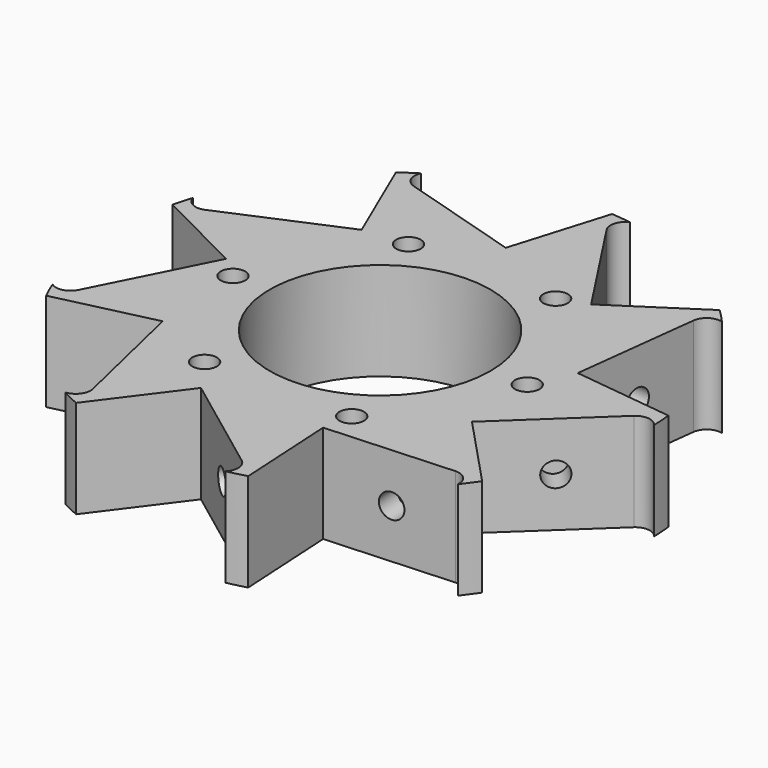
from build123d import *

# Parameters (mm, degrees)
F0_R      = 22.5
F1_DEPTH  = 20
F2_R      = 2.5
F3_DEPTH  = 20.001
F4_R      = 2.5
F5_DEPTH  = 5
F6_R      = 2.5
F7_DEPTH  = 5
F8_R      = 2.5
F9_DEPTH  = 5
F10_R     = 2.5
F11_DEPTH = 5
F12_R     = 2.5
F13_DEPTH = 5
F14_R     = 2.5
F15_DEPTH = 5
F16_R     = 2.5
F17_DEPTH = 5
F18_R     = 2.5
F19_DEPTH = 5
F20_R     = 2.5
F21_DEPTH = 5


# Not quite as in the source:
# - a feature names something its author has since deleted; it is built from what else it names


with BuildPart() as f1:
    # F0 (on Top) → F1 (new body)
    with BuildSketch(Plane.XY):
        with BuildLine():
            ThreePointArc((50, 2.2360679775), (52.3585771958, 2.9784933095), (54.4735576923, 1.6975017946))
            ThreePointArc((54.4735576923, 1.6975017946), (54.3740921627, 3.7024453378), (54.2008581475, 5.7023658309))
            Line((54.2008581475, 5.7023658309), (33.7982304406, 8.1353188741))
            Line((33.7982304406, 8.1353188741), (36.8649053656, 33.8523079329))
            ThreePointArc((36.8649053656, 33.8523079329), (38.1944585155, 35.9371029308), (40.6380330461, 36.3152897571))
            ThreePointArc((40.6380330461, 36.3152897571), (39.2730851622, 37.7872304071), (37.8548560942, 39.207905709))
            Line((37.8548560942, 39.207905709), (20.6616644432, 27.9570995731))
            Line((20.6616644432, 27.9570995731), (6.4803118028, 49.62867678))
            ThreePointArc((6.4803118028, 49.62867678), (6.1587282118, 52.0803426945), (7.7875210962, 53.9407500428))
            ThreePointArc((7.7875210962, 53.9407500428), (5.7957651426, 54.1909504107), (3.7961461645, 54.3676307585))
            Line((3.7961461645, 54.3676307585), (-2.1427239761, 34.6974426733))
            Line((-2.1427239761, 34.6974426733), (-26.9364916731, 42.1832362005))
            ThreePointArc((-26.9364916731, 42.1832362005), (-28.7587394689, 43.8546113028), (-28.7068585233, 46.3267338987))
            ThreePointArc((-28.7068585233, 46.3267338987), (-30.3934578, 45.2381224517), (-32.038822745, 44.0881371472))
            Line((-32.038822745, 44.0881371472), (-23.9445080332, 25.2024667275))
            Line((-23.9445080332, 25.2024667275), (-47.7494113294, 14.9997905883))
            ThreePointArc((-47.7494113294, 14.9997905883), (-50.2196733343, 15.1088198928), (-51.7689799985, 17.0359240992))
            ThreePointArc((-51.7689799985, 17.0359240992), (-52.3612440523, 15.1178742319), (-52.8824704203, 13.1793141796))
            Line((-52.8824704203, 13.1793141796), (-34.542390668, 3.9149765057))
            Line((-34.542390668, 3.9149765057), (-46.2198507491, -19.2022237443))
            ThreePointArc((-46.2198507491, -19.2022237443), (-48.1822639171, -20.7065562608), (-50.6078203843, -20.2261839196))
            ThreePointArc((-50.6078203843, -20.2261839196), (-49.8286222822, -22.0761953575), (-48.9818224627, -23.8962563644))
            Line((-48.9818224627, -23.8962563644), (-28.9775048134, -19.2043747332))
            Line((-28.9775048134, -19.2043747332), (-23.0635083269, -44.419304178))
            ThreePointArc((-23.0635083269, -44.419304178), (-23.5998377269, -46.8331046123), (-25.766699169, -48.0242356934))
            ThreePointArc((-25.766699169, -48.0242356934), (-23.9806343627, -48.9405677895), (-22.1620354025, -49.7905029782))
            Line((-22.1620354025, -49.7905029782), (-9.8537224074, -33.3377856016))
            Line((-9.8537224074, -33.3377856016), (10.8845059639, -48.8520985212))
            ThreePointArc((10.8845059639, -48.8520985212), (12.0252148188, -51.0459228237), (11.1309469524, -53.3512138563))
            ThreePointArc((11.1309469524, -53.3512138563), (13.0881588901, -52.905104639), (15.0276143261, -52.3872198887))
            Line((15.0276143261, -52.3872198887), (13.8807262249, -31.8720760788))
            Line((13.8807262249, -31.8720760788), (39.7395389463, -30.4264530357))
            ThreePointArc((39.7395389463, -30.4264530357), (42.0235357053, -31.3737864336), (42.8202992881, -33.7145661232))
            ThreePointArc((42.8202992881, -33.7145661232), (44.0328571396, -32.1147550532), (45.1856762982, -30.4713743942))
            Line((45.1856762982, -30.4713743942), (31.1202287894, -15.49306794))
            Line((31.1202287894, -15.49306794), (50, 2.2360679775))
        make_face()
        Circle(F0_R, mode=Mode.SUBTRACT)
    extrude(amount=F1_DEPTH)

    # F2 (on face) → F3 (cut, through all)
    with BuildSketch(Plane.XY.offset(20)):
        with Locations((15, 25.9807621135)):
            Circle(F2_R)
        with BuildLine():
            ThreePointArc((32.5, 0), (30, 2.5), (27.5, 0))
            ThreePointArc((27.5, 0), (30, -2.5), (32.5, 0))
        make_face()
        with Locations((15, -25.9807621135)):
            Circle(F2_R)
        with Locations((-15, -25.9807621135)):
            Circle(F2_R)
        with Locations((-30, 0)):
            Circle(F2_R)
        with Locations((-15, 25.9807621135)):
            Circle(F2_R)
    extrude(amount=-F3_DEPTH, mode=Mode.SUBTRACT)

    # F4 (on face) → F5 (cut)
    with BuildSketch(Plane(origin=(32.3678514777, -3.8597706083, 0), x_dir=(0.1184081423, 0.9929650104, 0), z_dir=(0.9929650104, -0.1184081423, 0))):
        with Locations((25.4792622567, 10)):
            Circle(F4_R)
    extrude(amount=-F5_DEPTH, mode=Mode.SUBTRACT)

    # F6 (on face) → F7 (cut)
    with BuildSketch(Plane(origin=(27.2762254834, 17.8488980559, 0), x_dir=(-0.5475597061, 0.8367666151, 0), z_dir=(0.8367666151, 0.5475597061, 0))):
        with Locations((25.4792622567, 10)):
            Circle(F6_R)
    extrude(amount=-F7_DEPTH, mode=Mode.SUBTRACT)

    # F8 (on face) → F9 (cut)
    with BuildSketch(Plane(origin=(9.421750444, 31.2058689513, 0), x_dir=(-0.9573182826, 0.289035821, 0), z_dir=(0.289035821, 0.9573182826, 0))):
        with Locations((25.4792622567, 10)):
            Circle(F8_R)
    extrude(amount=-F9_DEPTH, mode=Mode.SUBTRACT)

    # F10 (on face) → F11 (cut)
    with BuildSketch(Plane(origin=(-12.8412663393, 29.9612669498, 0), x_dir=(-0.9191369952, -0.393938046, 0), z_dir=(-0.393938046, 0.9191369952, 0))):
        with Locations((25.4792622567, 10)):
            Circle(F10_R)
    extrude(amount=-F11_DEPTH, mode=Mode.SUBTRACT)

    # F12 (on face) → F13 (cut)
    with BuildSketch(Plane(origin=(-29.0957118877, 14.6974551601, 0), x_dir=(-0.4508812927, -0.8925839232, 0), z_dir=(-0.8925839232, 0.4508812927, 0))):
        with Locations((25.4792622567, 10)):
            Circle(F12_R)
    extrude(amount=-F13_DEPTH, mode=Mode.SUBTRACT)

    # F14 (on face) → F15 (cut)
    with BuildSketch(Plane(origin=(-31.735950481, -7.4434592431, 0), x_dir=(0.2283467777, -0.9735798627, 0), z_dir=(-0.9735798627, -0.2283467777, 0))):
        with Locations((25.4792622567, 10)):
            Circle(F14_R)
    extrude(amount=-F15_DEPTH, mode=Mode.SUBTRACT)

    # F16 (on face) → F17 (cut)
    with BuildSketch(Plane(origin=(-19.5265851384, -26.1014963415, 0), x_dir=(0.8007288529, -0.5990269644, 0), z_dir=(-0.5990269644, -0.8007288529, 0))):
        with Locations((25.4792622567, 10)):
            Circle(F16_R)
    extrude(amount=-F17_DEPTH, mode=Mode.SUBTRACT)

    # F18 (on face) → F19 (cut)
    with BuildSketch(Plane(origin=(1.8194864043, -32.546353216, 0), x_dir=(0.9984409988, 0.055817308, 0), z_dir=(0.055817308, -0.9984409988, 0))):
        with Locations((25.4792622567, 10)):
            Circle(F18_R)
    extrude(amount=-F19_DEPTH, mode=Mode.SUBTRACT)

    # F20 (on face) → F21 (cut)
    with BuildSketch(Plane(origin=(22.314200037, -23.7624097082, 0), x_dir=(0.7289715049, 0.6845440417, 0), z_dir=(0.6845440417, -0.7289715049, 0))):
        with Locations((25.4792622567, 10)):
            Circle(F20_R)
    extrude(amount=-F21_DEPTH, mode=Mode.SUBTRACT)


solid = f1.part
